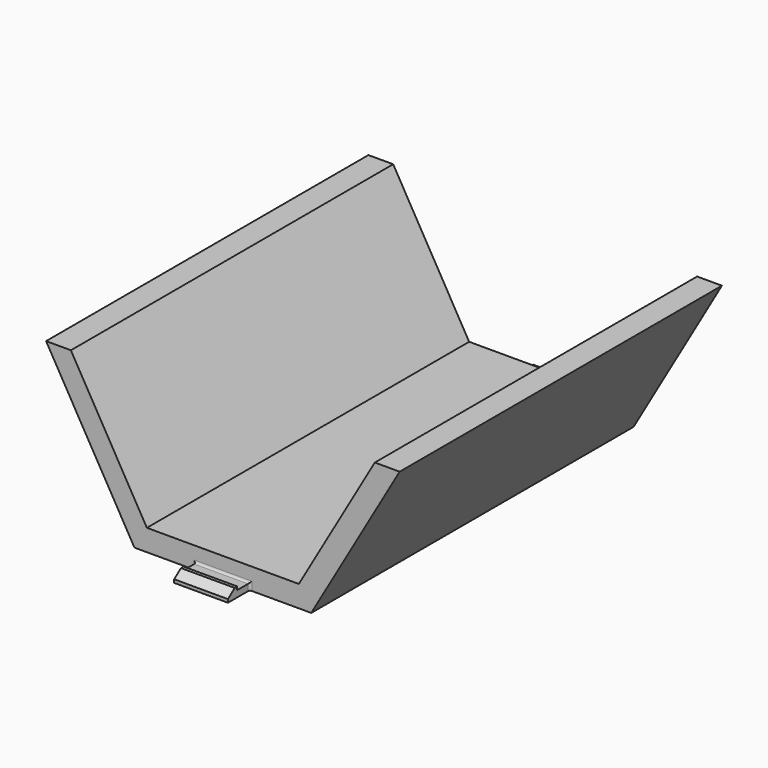
from build123d import *

# Parameters (mm, degrees)
F1_DEPTH = 47.625
F3_DEPTH = 6.35
F4_R     = 0.508


# Not quite as in the source:
# - a pattern or mirror of a feature is missing from the dataset's text; its kind, count and spacing are read off the source's solid


with BuildPart() as f1:
    # F0 (on Front) → F1 (new body, symmetric)
    with BuildSketch(Plane.XZ):
        Polygon((20.8971929933, 0), (41.7943859866, 36.195), (35.9285072517, 36.195), (17.9642536258, 5.08), (-17.9642536258, 5.08), (-35.9285072517, 36.195), (-41.7943859866, 36.195), (-20.8971929933, 0), align=None)
    extrude(amount=F1_DEPTH, both=True)

    # F2 (on Right) → F3 (join, symmetric)
    with BuildSketch(Plane.YZ):
        Polygon((-47.625, 1.524), (-51.308, 1.524), (-51.308, 2.286), (-52.07, 2.286), (-54.0561154682, 0.762), (-54.0561154682, 0), (-47.625, 0), align=None)
    f3 = extrude(amount=F3_DEPTH, both=True)

    # F3_copies: F3 across plane
    add(f3.mirror(Plane.ZX))

    # F4
    f4_edges = [f1.edges().sort_by_distance(p)[0] for p in [
        (-6.35, -47.625, 0.762),
        (6.35, -47.625, 0.762),
        (0, -47.625, 1.524),
        (6.35, 47.625, 0.762),
        (0, 47.625, 1.524),
        (-6.35, 47.625, 0.762),
    ]]
    fillet(f4_edges, radius=F4_R)


solid = f1.part
